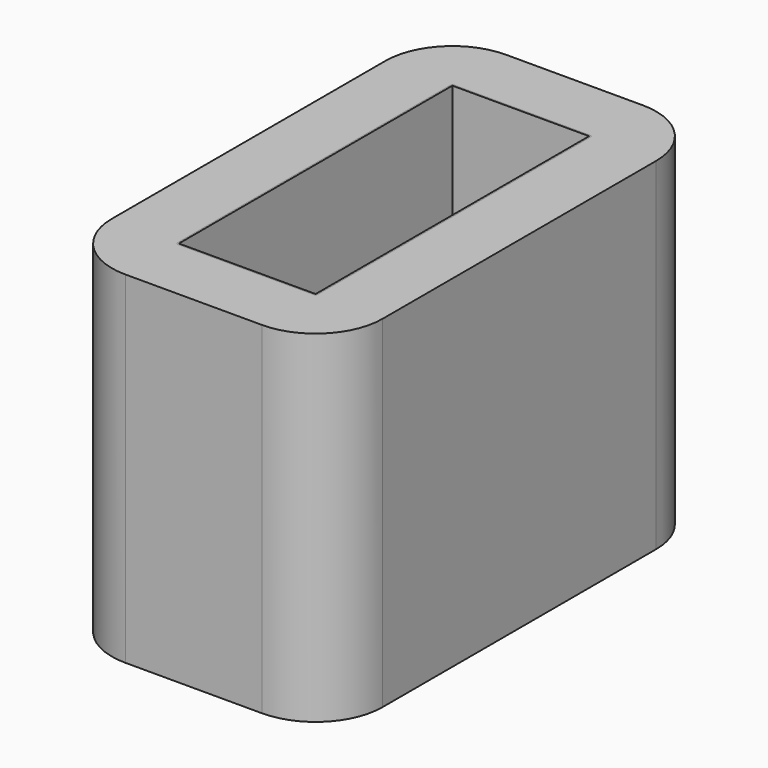
from build123d import *

# Parameters (mm, degrees)
F4_W      = 120.7008
F4_H      = 212.1408
F5_DEPTH  = 152.4
F6_R      = 29.8704
F7_W      = 62.484
F7_H      = 153.924
F8_DEPTH  = 152.4
F9_W      = 62.484
F9_H      = 153.924
F10_DEPTH = 152.4
F11_W     = 60.96
F11_H     = 152.4
F12_DEPTH = 152.4
F13_R     = 0.762
F14_R     = 0.762


with BuildPart() as f5:
    # F4 (on Top) → F5 (new body)
    with BuildSketch(Plane.XY):
        Rectangle(F4_W, F4_H)
    extrude(amount=-F5_DEPTH)

    # F6
    f6_edges = [f5.edges().sort_by_distance(p)[0] for p in [
        (-60.3504, 106.0704, -76.2),
        (60.3504, 106.0704, -76.2),
        (60.3504, -106.0704, -76.2),
        (-60.3504, -106.0704, -76.2),
    ]]
    fillet(f6_edges, radius=F6_R)

    # F7 (on face) → F8 (cut)
    with BuildSketch(Plane.XY):
        Rectangle(F7_W, F7_H)
    extrude(amount=-F8_DEPTH, mode=Mode.SUBTRACT)

    # F14
    f14_edges = [f5.edges().sort_by_distance(p)[0] for p in [
        (-31.242, 76.962, -76.2),
        (-31.242, -76.962, -76.2),
        (31.242, -76.962, -76.2),
        (31.242, 76.962, -76.2),
    ]]
    fillet(f14_edges, radius=F14_R)


with BuildPart() as f10:
    # F9 (on face) → F10 (new body)
    with BuildSketch(Plane.XY):
        Rectangle(F9_W, F9_H)
    extrude(amount=-F10_DEPTH)

    # F11 (on face) → F12 (cut)
    with BuildSketch(Plane.XY):
        Rectangle(F11_W, F11_H)
    extrude(amount=-F12_DEPTH, mode=Mode.SUBTRACT)

    # F13
    f13_edges = [f10.edges().sort_by_distance(p)[0] for p in [
        (-31.242, 76.962, -76.2),
        (31.242, 76.962, -76.2),
        (31.242, -76.962, -76.2),
        (-31.242, -76.962, -76.2),
    ]]
    fillet(f13_edges, radius=F13_R)


solid = Compound([f5.part, f10.part])
